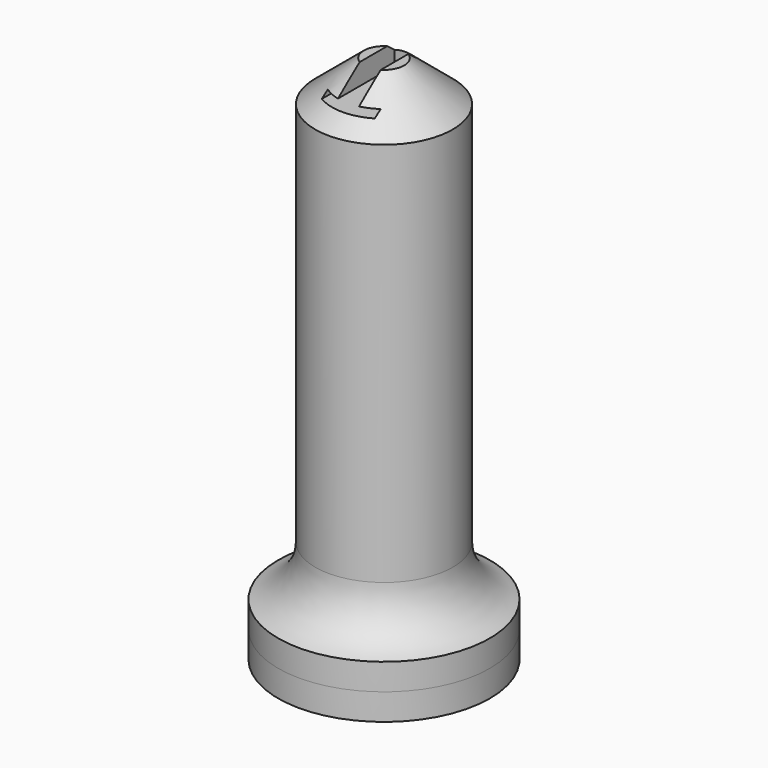
from build123d import *

# Parameters (mm, degrees)
F0_W     = 2.5
F0_H     = 2.5
F0_W_2   = 3.5
F3_W     = 1.9934664722
F3_H     = 2
F3_H_2   = 0.5
F3_W_2   = 1.5032667639
F4_DEPTH = 27.5
F5_R     = 10
F5_R_2   = 7.25
F6_DEPTH = 2.5


# Not quite as in the source:
# - a fillet or chamfer that OpenCascade refuses, or shapes differently, is made with other operations: its cross-section is extruded or revolved along the edge and cut away or added


with BuildPart() as f1:
    # F0 (on Front) → F1 (revolve)
    with BuildSketch(Plane.XZ):
        Polygon((-6.5, 0), (-4, 0), (-4, 40), (-1, 42.5), (0, 42.5), (0, 45), (-1.905124838, 45), (-6.5, 41.170937365), align=None)
        with Locations((-5.25, -1.25)):
            Rectangle(F0_W, F0_H)
        with Locations((-8.25, -1.25)):
            Rectangle(F0_W_2, F0_H)
    revolve(axis=Axis((0, 0, 20), (0, 0, 1)))

    # F3 (on offset) → F4 (cut)
    with BuildSketch(Plane.XZ.offset(25)):
        with Locations((0, 44)):
            Rectangle(F3_W, F3_H)
        with Locations((0, 42.75)):
            Rectangle(F3_W, F3_H_2)
        with Locations((-1.7483666181, 42.75)):
            Rectangle(F3_W_2, F3_H_2)
        with Locations((1.7483666181, 42.75)):
            Rectangle(F3_W_2, F3_H_2)
    extrude(amount=-F4_DEPTH, mode=Mode.SUBTRACT)

    # F5 (on face) → F6 (join)
    with BuildSketch(Plane(origin=(0, 0, -2.5), x_dir=(1, 0, 0), z_dir=(0, 0, -1))):
        Circle(F5_R)
        Circle(F5_R_2, mode=Mode.SUBTRACT)
    extrude(amount=F6_DEPTH)

    # F7: fillet of radius 5 on 1 edges, made by hand

    # F7_s1 → F7_t2 (revolve)
    with BuildSketch(Plane.XZ):
        with BuildLine():
            ThreePointArc((-6.5, 4.7696960071), (-7.4688711259, 1.8116561155), (-10, 0))
            Line((-10, 0), (-6.5, 0))
            Line((-6.5, 0), (-6.5, 4.7696960071))
        make_face()
    revolve(axis=Axis((0, 0, 0), (0, 0, 1)))


solid = f1.part
